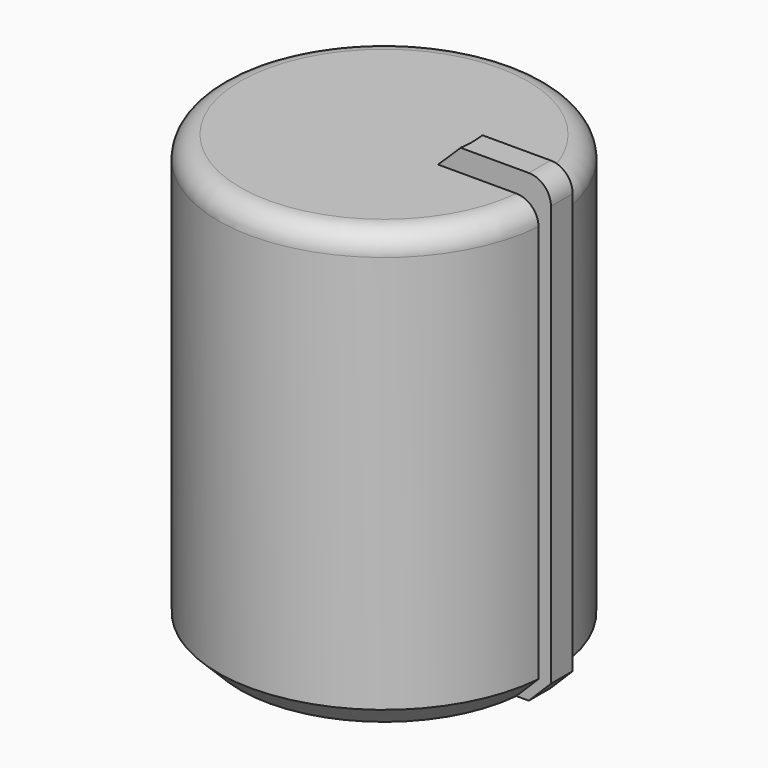
from build123d import *

# Parameters (mm, degrees)
F1_DEPTH = 20
F2_DEPTH = 21
F3_DEPTH = 18
F4_DEPTH = 10
F10_R    = 1
F6_SIZE  = 0.99999
F7_SIZE  = 1
F8_SIZE  = 1
F9_SIZE  = 2.5


# Not quite as in the source:
# - a fillet or chamfer that OpenCascade refuses, or shapes differently, is made with other operations: its cross-section is extruded or revolved along the edge and cut away or added
# - a fillet or chamfer is up to 0.001 mm smaller than in the source, because OpenCascade refuses the exact size


with BuildPart() as f1:
    # F0 (on Top) → F1 (new body)
    with BuildSketch(Plane.XY):
        with BuildLine():
            ThreePointArc((3, 0), (2.9840537841, 0.308906157), (2.9363846575, 0.6145283911))
            Line((2.9363846575, 0.6145283911), (2.9363846575, -0.6145283911))
            ThreePointArc((2.9363846575, -0.6145283911), (2.9840537841, -0.308906157), (3, 0))
        make_face()
        with BuildLine():
            Line((5.5474227354, 0.6145283911), (7.4747812581, 0.6145283911))
            ThreePointArc((7.4747812581, 0.6145283911), (-7.5, 0), (7.4747812581, -0.6145283911))
            Line((7.4747812581, -0.6145283911), (5.5474227354, -0.6145283911))
            ThreePointArc((5.5474227354, -0.6145283911), (-5.5813568376, 0), (5.5474227354, 0.6145283911))
        make_face()
        with BuildLine():
            Line((2.9363846575, 0.6145283911), (5.5474227354, 0.6145283911))
            ThreePointArc((5.5474227354, 0.6145283911), (-5.5813568376, 0), (5.5474227354, -0.6145283911))
            Line((5.5474227354, -0.6145283911), (2.9363846575, -0.6145283911))
            ThreePointArc((2.9363846575, -0.6145283911), (-3, 0), (2.9363846575, 0.6145283911))
        make_face()
        with BuildLine():
            Line((2.9363846575, -0.6145283911), (2.9363846575, 0.6145283911))
            ThreePointArc((2.9363846575, 0.6145283911), (-3, 0), (2.9363846575, -0.6145283911))
        make_face()
        with BuildLine():
            ThreePointArc((7.4747812581, -0.6145283911), (7.4936926624, -0.3075228156), (7.5, 0))
            ThreePointArc((7.5, 0), (7.4936926624, 0.3075228156), (7.4747812581, 0.6145283911))
            Line((7.4747812581, 0.6145283911), (5.5474227354, 0.6145283911))
            ThreePointArc((5.5474227354, 0.6145283911), (5.5728668548, 0.3077322971), (5.5813568376, 0))
            ThreePointArc((5.5813568376, 0), (5.5728668548, -0.3077322971), (5.5474227354, -0.6145283911))
            Line((5.5474227354, -0.6145283911), (7.4747812581, -0.6145283911))
        make_face()
        with BuildLine():
            ThreePointArc((5.5813568376, 0), (5.5728668548, 0.3077322971), (5.5474227354, 0.6145283911))
            Line((5.5474227354, 0.6145283911), (2.9363846575, 0.6145283911))
            ThreePointArc((2.9363846575, 0.6145283911), (2.9840537841, 0.308906157), (3, 0))
            ThreePointArc((3, 0), (2.9840537841, -0.308906157), (2.9363846575, -0.6145283911))
            Line((2.9363846575, -0.6145283911), (5.5474227354, -0.6145283911))
            ThreePointArc((5.5474227354, -0.6145283911), (5.5728668548, -0.3077322971), (5.5813568376, 0))
        make_face()
    extrude(amount=F1_DEPTH)

    # F0 (on Top) → F2 (join)
    with BuildSketch(Plane.XY):
        with BuildLine():
            ThreePointArc((7.4747812581, 0.6145283911), (7.4936926624, 0.3075228156), (7.5, 0))
            ThreePointArc((7.5, 0), (7.4936926624, -0.3075228156), (7.4747812581, -0.6145283911))
            Line((7.4747812581, -0.6145283911), (8.0371221235, -0.6145283911))
            Line((8.0371221235, -0.6145283911), (8.0371221235, 0.6145283911))
            Line((8.0371221235, 0.6145283911), (7.4747812581, 0.6145283911))
        make_face()
        with BuildLine():
            ThreePointArc((7.4747812581, -0.6145283911), (7.4936926624, -0.3075228156), (7.5, 0))
            ThreePointArc((7.5, 0), (7.4936926624, 0.3075228156), (7.4747812581, 0.6145283911))
            Line((7.4747812581, 0.6145283911), (5.5474227354, 0.6145283911))
            ThreePointArc((5.5474227354, 0.6145283911), (5.5728668548, 0.3077322971), (5.5813568376, 0))
            ThreePointArc((5.5813568376, 0), (5.5728668548, -0.3077322971), (5.5474227354, -0.6145283911))
            Line((5.5474227354, -0.6145283911), (7.4747812581, -0.6145283911))
        make_face()
        with BuildLine():
            ThreePointArc((5.5813568376, 0), (5.5728668548, 0.3077322971), (5.5474227354, 0.6145283911))
            Line((5.5474227354, 0.6145283911), (2.9363846575, 0.6145283911))
            ThreePointArc((2.9363846575, 0.6145283911), (2.9840537841, 0.308906157), (3, 0))
            ThreePointArc((3, 0), (2.9840537841, -0.308906157), (2.9363846575, -0.6145283911))
            Line((2.9363846575, -0.6145283911), (5.5474227354, -0.6145283911))
            ThreePointArc((5.5474227354, -0.6145283911), (5.5728668548, -0.3077322971), (5.5813568376, 0))
        make_face()
    extrude(amount=F2_DEPTH)

    # F0 (on Top) → F3 (cut)
    with BuildSketch(Plane.XY):
        with BuildLine():
            Line((2.9363846575, -0.6145283911), (2.9363846575, 0.6145283911))
            ThreePointArc((2.9363846575, 0.6145283911), (-3, 0), (2.9363846575, -0.6145283911))
        make_face()
        with BuildLine():
            ThreePointArc((3, 0), (2.9840537841, 0.308906157), (2.9363846575, 0.6145283911))
            Line((2.9363846575, 0.6145283911), (2.9363846575, -0.6145283911))
            ThreePointArc((2.9363846575, -0.6145283911), (2.9840537841, -0.308906157), (3, 0))
        make_face()
    extrude(amount=F3_DEPTH, mode=Mode.SUBTRACT)

    # F0 (on Top) → F4 (cut)
    with BuildSketch(Plane.XY):
        with BuildLine():
            Line((2.9363846575, 0.6145283911), (5.5474227354, 0.6145283911))
            ThreePointArc((5.5474227354, 0.6145283911), (-5.5813568376, 0), (5.5474227354, -0.6145283911))
            Line((5.5474227354, -0.6145283911), (2.9363846575, -0.6145283911))
            ThreePointArc((2.9363846575, -0.6145283911), (-3, 0), (2.9363846575, 0.6145283911))
        make_face()
        with BuildLine():
            ThreePointArc((5.5813568376, 0), (5.5728668548, 0.3077322971), (5.5474227354, 0.6145283911))
            Line((5.5474227354, 0.6145283911), (2.9363846575, 0.6145283911))
            ThreePointArc((2.9363846575, 0.6145283911), (2.9840537841, 0.308906157), (3, 0))
            ThreePointArc((3, 0), (2.9840537841, -0.308906157), (2.9363846575, -0.6145283911))
            Line((2.9363846575, -0.6145283911), (5.5474227354, -0.6145283911))
            ThreePointArc((5.5474227354, -0.6145283911), (5.5728668548, -0.3077322971), (5.5813568376, 0))
        make_face()
    extrude(amount=F4_DEPTH, mode=Mode.SUBTRACT)

    # F10
    f10_edges = [f1.edges().sort_by_distance(p)[0] for p in [
        (-7.5, 0, 20),
        (8.037122, 0, 21),
    ]]
    fillet(f10_edges, radius=F10_R)

    # F5: chamfer of 3 on 1 edges, made by hand

    # F5_s1 → F5_t2 (revolve)
    with BuildSketch(Plane(origin=(0, 0, 0), x_dir=(0, 0, 1), z_dir=(-0.204842797, -0.9787948858, 0))):
        Polygon((15, -3), (18, 0), (18, -3), align=None)
    revolve(axis=Axis((0, 0, 18), (0, 0, 1)))

    # F6 (size 1 in the source; OpenCascade refuses exactly that, so slightly less here)
    f6_edges = [f1.edges().sort_by_distance(p)[0] for p in [
        (3, 0, 21),
    ]]
    chamfer(f6_edges, length=F6_SIZE)

    # F7
    f7_edges = [f1.edges().sort_by_distance(p)[0] for p in [
        (-7.5, 0, 0),
    ]]
    chamfer(f7_edges, length=F7_SIZE)

    # F8
    f8_edges = [f1.edges().sort_by_distance(p)[0] for p in [
        (8.037122, 0, 0),
    ]]
    chamfer(f8_edges, length=F8_SIZE)

    # F9
    f9_edges = [f1.edges().sort_by_distance(p)[0] for p in [
        (-5.547423, 0.614528, 10),
    ]]
    chamfer(f9_edges, length=F9_SIZE)


solid = f1.part
